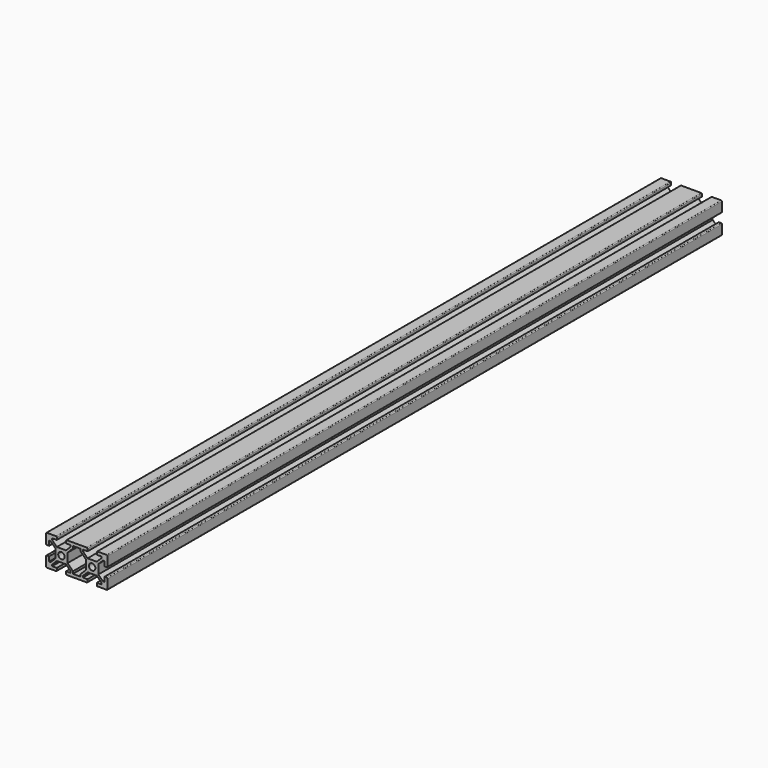
from build123d import *

# Parameters (mm, degrees)
F1_DEPTH = 500
F2_R     = 0.5


with BuildPart() as f1:
    # F0 (on Front) → F1 (new body)
    with BuildSketch(Plane.XZ):
        Polygon((-250.682858482, 19.2996120907), (-257.682858482, 19.2996120907), (-257.682858482, 12.2996120907), (-255.682858482, 12.2996120907), (-255.682858482, 15.2996120907), (-254.682858482, 15.2996120907), (-251.682858482, 12.2996120907), (-251.682858482, 13.2996120907), (-250.682858482, 13.2996120907), (-253.682858482, 16.2996120907), (-253.682858482, 17.2996120907), (-250.682858482, 17.2996120907), align=None)
        Polygon((-237.682858482, 19.2996120907), (-244.682858482, 19.2996120907), (-244.682858482, 17.2996120907), (-241.682858482, 17.2996120907), (-241.682858482, 16.2996120907), (-244.682858482, 13.2996120907), (-243.682858482, 13.2996120907), (-243.682858482, 12.2996120907), (-240.182858482, 15.7996120907), (-240.182858482, 17.2996120907), (-237.682858482, 17.2996120907), align=None)
        Polygon((-230.682858482, 19.2996120907), (-237.682858482, 19.2996120907), (-237.682858482, 17.2996120907), (-235.182858482, 17.2996120907), (-235.182858482, 15.7996120907), (-231.682858482, 12.2996120907), (-231.682858482, 13.2996120907), (-230.682858482, 13.2996120907), (-233.682858482, 16.2996120907), (-233.682858482, 17.2996120907), (-230.682858482, 17.2996120907), align=None)
        Polygon((-255.682858482, 6.2996120907), (-257.682858482, 6.2996120907), (-257.682858482, -0.7003879093), (-250.682858482, -0.7003879093), (-250.682858482, 1.2996120907), (-253.682858482, 1.2996120907), (-253.682858482, 2.2996120907), (-250.682858482, 5.2996120907), (-251.682858482, 5.2996120907), (-251.682858482, 6.2996120907), (-254.682858482, 3.2996120907), (-255.682858482, 3.2996120907), align=None)
        with BuildLine():
            ThreePointArc((-247.6828584684, 5.2996120907), (-250.5112856019, 6.4711849611), (-251.682858482, 9.2996120907))
            Line((-251.682858482, 9.2996120907), (-251.682858482, 6.2996120907))
            Line((-251.682858482, 6.2996120907), (-251.682858482, 5.2996120907))
            Line((-251.682858482, 5.2996120907), (-250.682858482, 5.2996120907))
            Line((-250.682858482, 5.2996120907), (-247.6828584684, 5.2996120907))
        make_face()
        with BuildLine():
            Line((-251.682858482, 12.2996120907), (-251.682858482, 9.2996120907))
            ThreePointArc((-251.682858482, 9.2996120907), (-250.5112856067, 12.1280392154), (-247.682858482, 13.2996120907))
            Line((-247.682858482, 13.2996120907), (-250.682858482, 13.2996120907))
            Line((-250.682858482, 13.2996120907), (-251.682858482, 13.2996120907))
            Line((-251.682858482, 13.2996120907), (-251.682858482, 12.2996120907))
        make_face()
        with BuildLine():
            Line((-249.782858482, 9.2996120907), (-251.682858482, 9.2996120907))
            ThreePointArc((-251.682858482, 9.2996120907), (-250.5112856019, 6.4711849611), (-247.6828584684, 5.2996120907))
            ThreePointArc((-247.6828584684, 5.2996120907), (-244.8544313524, 6.4711849708), (-243.682858482, 9.2996120907))
            Line((-243.682858482, 9.2996120907), (-245.582858482, 9.2996120907))
            ThreePointArc((-245.582858482, 9.2996120907), (-247.682858482, 7.1996120907), (-249.782858482, 9.2996120907))
        make_face()
        with BuildLine():
            ThreePointArc((-247.682858482, 13.2996120907), (-250.5112856067, 12.1280392154), (-251.682858482, 9.2996120907))
            Line((-251.682858482, 9.2996120907), (-249.782858482, 9.2996120907))
            ThreePointArc((-249.782858482, 9.2996120907), (-247.682858482, 11.3996120907), (-245.582858482, 9.2996120907))
            Line((-245.582858482, 9.2996120907), (-243.682858482, 9.2996120907))
            ThreePointArc((-243.682858482, 9.2996120907), (-244.8544313573, 12.1280392154), (-247.682858482, 13.2996120907))
        make_face()
        Polygon((-217.682858482, 19.2996120907), (-224.682858482, 19.2996120907), (-224.682858482, 17.2996120907), (-221.682858482, 17.2996120907), (-221.682858482, 16.2996120907), (-224.682858482, 13.2996120907), (-223.682858482, 13.2996120907), (-223.682858482, 12.2996120907), (-220.682858482, 15.2996120907), (-219.682858482, 15.2996120907), (-219.682858482, 12.2996120907), (-217.682858482, 12.2996120907), align=None)
        with BuildLine():
            Line((-244.682858482, 13.2996120907), (-247.682858482, 13.2996120907))
            ThreePointArc((-247.682858482, 13.2996120907), (-244.8544313573, 12.1280392154), (-243.682858482, 9.2996120907))
            Line((-243.682858482, 9.2996120907), (-243.682858482, 12.2996120907))
            Line((-243.682858482, 12.2996120907), (-243.682858482, 13.2996120907))
            Line((-243.682858482, 13.2996120907), (-244.682858482, 13.2996120907))
        make_face()
        with BuildLine():
            ThreePointArc((-243.682858482, 9.2996120907), (-244.8544313524, 6.4711849708), (-247.6828584684, 5.2996120907))
            Line((-247.6828584684, 5.2996120907), (-244.682858482, 5.2996120907))
            Line((-244.682858482, 5.2996120907), (-243.682858482, 5.2996120907))
            Line((-243.682858482, 5.2996120907), (-243.682858482, 6.2996120907))
            Line((-243.682858482, 6.2996120907), (-243.682858482, 9.2996120907))
        make_face()
        with BuildLine():
            ThreePointArc((-227.682858482, 5.2996120907), (-230.5112856067, 6.4711849659), (-231.682858482, 9.2996120907))
            Line((-231.682858482, 9.2996120907), (-231.682858482, 6.2996120907))
            Line((-231.682858482, 6.2996120907), (-231.682858482, 5.2996120907))
            Line((-231.682858482, 5.2996120907), (-230.682858482, 5.2996120907))
            Line((-230.682858482, 5.2996120907), (-227.682858482, 5.2996120907))
        make_face()
        with BuildLine():
            Line((-231.682858482, 12.2996120907), (-231.682858482, 9.2996120907))
            ThreePointArc((-231.682858482, 9.2996120907), (-230.5112856067, 12.1280392154), (-227.682858482, 13.2996120907))
            Line((-227.682858482, 13.2996120907), (-230.682858482, 13.2996120907))
            Line((-230.682858482, 13.2996120907), (-231.682858482, 13.2996120907))
            Line((-231.682858482, 13.2996120907), (-231.682858482, 12.2996120907))
        make_face()
        with BuildLine():
            Line((-229.782858482, 9.2996120907), (-231.682858482, 9.2996120907))
            ThreePointArc((-231.682858482, 9.2996120907), (-230.5112856067, 6.4711849659), (-227.682858482, 5.2996120907))
            ThreePointArc((-227.682858482, 5.2996120907), (-224.8544313573, 6.4711849659), (-223.682858482, 9.2996120907))
            Line((-223.682858482, 9.2996120907), (-225.582858482, 9.2996120907))
            ThreePointArc((-225.582858482, 9.2996120907), (-227.682858482, 7.1996120907), (-229.782858482, 9.2996120907))
        make_face()
        with BuildLine():
            ThreePointArc((-227.682858482, 13.2996120907), (-230.5112856067, 12.1280392154), (-231.682858482, 9.2996120907))
            Line((-231.682858482, 9.2996120907), (-229.782858482, 9.2996120907))
            ThreePointArc((-229.782858482, 9.2996120907), (-227.682858482, 11.3996120907), (-225.582858482, 9.2996120907))
            Line((-225.582858482, 9.2996120907), (-223.682858482, 9.2996120907))
            ThreePointArc((-223.682858482, 9.2996120907), (-224.8544313573, 12.1280392154), (-227.682858482, 13.2996120907))
        make_face()
        Polygon((-235.182858482, 1.2996120907), (-237.682858482, 1.2996120907), (-237.682858482, -0.7003879093), (-230.682858482, -0.7003879093), (-230.682858482, 1.2996120907), (-233.682858482, 1.2996120907), (-233.682858482, 2.2996120907), (-230.682858482, 5.2996120907), (-231.682858482, 5.2996120907), (-231.682858482, 6.2996120907), (-235.182858482, 2.7996120907), align=None)
        Polygon((-237.682858482, -0.7003879093), (-237.682858482, 1.2996120907), (-240.182858482, 1.2996120907), (-240.182858482, 2.7996120907), (-243.682858482, 6.2996120907), (-243.682858482, 5.2996120907), (-244.682858482, 5.2996120907), (-241.682858482, 2.2996120907), (-241.682858482, 1.2996120907), (-244.682858482, 1.2996120907), (-244.682858482, -0.7003879093), align=None)
        with BuildLine():
            Line((-224.682858482, 13.2996120907), (-227.682858482, 13.2996120907))
            ThreePointArc((-227.682858482, 13.2996120907), (-224.8544313573, 12.1280392154), (-223.682858482, 9.2996120907))
            Line((-223.682858482, 9.2996120907), (-223.682858482, 12.2996120907))
            Line((-223.682858482, 12.2996120907), (-223.682858482, 13.2996120907))
            Line((-223.682858482, 13.2996120907), (-224.682858482, 13.2996120907))
        make_face()
        with BuildLine():
            ThreePointArc((-223.682858482, 9.2996120907), (-224.8544313573, 6.4711849659), (-227.682858482, 5.2996120907))
            Line((-227.682858482, 5.2996120907), (-224.682858482, 5.2996120907))
            Line((-224.682858482, 5.2996120907), (-223.682858482, 5.2996120907))
            Line((-223.682858482, 5.2996120907), (-223.682858482, 6.2996120907))
            Line((-223.682858482, 6.2996120907), (-223.682858482, 9.2996120907))
        make_face()
        Polygon((-223.682858482, 5.2996120907), (-224.682858482, 5.2996120907), (-221.682858482, 2.2996120907), (-221.682858482, 1.2996120907), (-224.682858482, 1.2996120907), (-224.682858482, -0.7003879093), (-217.682858482, -0.7003879093), (-217.682858482, 6.2996120907), (-219.682858482, 6.2996120907), (-219.682858482, 3.2996120907), (-220.682858482, 3.2996120907), (-223.682858482, 6.2996120907), align=None)
    extrude(amount=F1_DEPTH)

    # F2
    f2_edges = [f1.edges().sort_by_distance(p)[0] for p in [
        (-257.682858, -250, 19.299612),
        (-250.682858, -250, 19.299612),
        (-244.682858, -250, 19.299612),
        (-230.682858, -250, 19.299612),
        (-224.682858, -250, 19.299612),
        (-217.682858, -250, 19.299612),
        (-217.682858, -250, 12.299612),
        (-217.682858, -250, 6.299612),
        (-217.682858, -250, -0.700388),
        (-230.682858, -250, -0.700388),
        (-250.682858, -250, -0.700388),
        (-257.682858, -250, 6.299612),
        (-257.682858, -250, 12.299612),
        (-257.682858, -250, -0.700388),
        (-244.682858, -250, -0.700388),
        (-224.682858, -250, -0.700388),
    ]]
    fillet(f2_edges, radius=F2_R)


solid = f1.part
